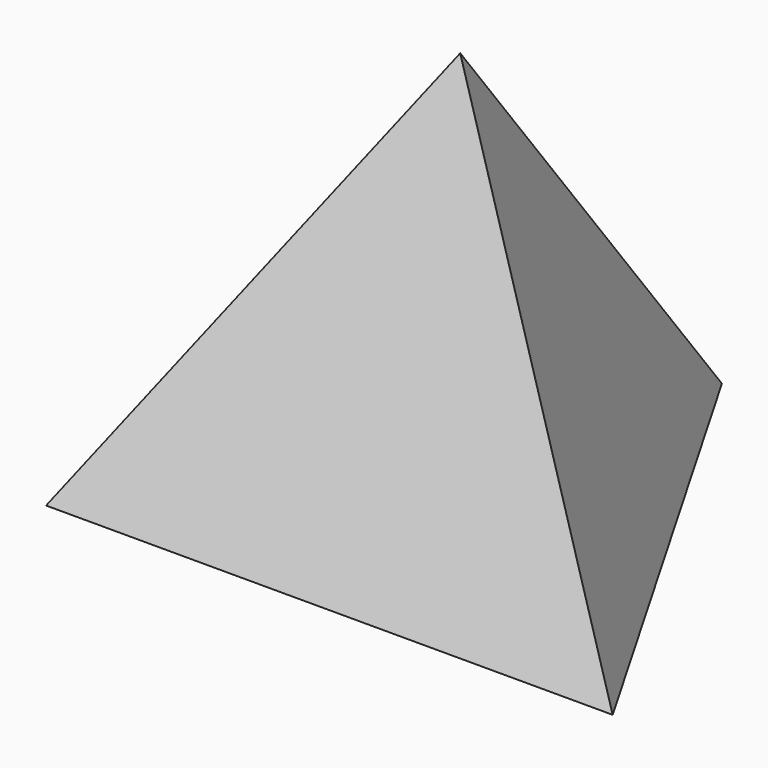
from build123d import *

# Parameters (mm, degrees)
F1_DEPTH = 50.8
F1_TAPER = 21.1


with BuildPart() as f1:
    # F0 (on Top) → F1 (new body)
    with BuildSketch(Plane.XY):
        Polygon((27.496307, -15.875), (0, 31.75), (-27.496307, -15.875), align=None)
    extrude(amount=F1_DEPTH, taper=F1_TAPER)


solid = f1.part
